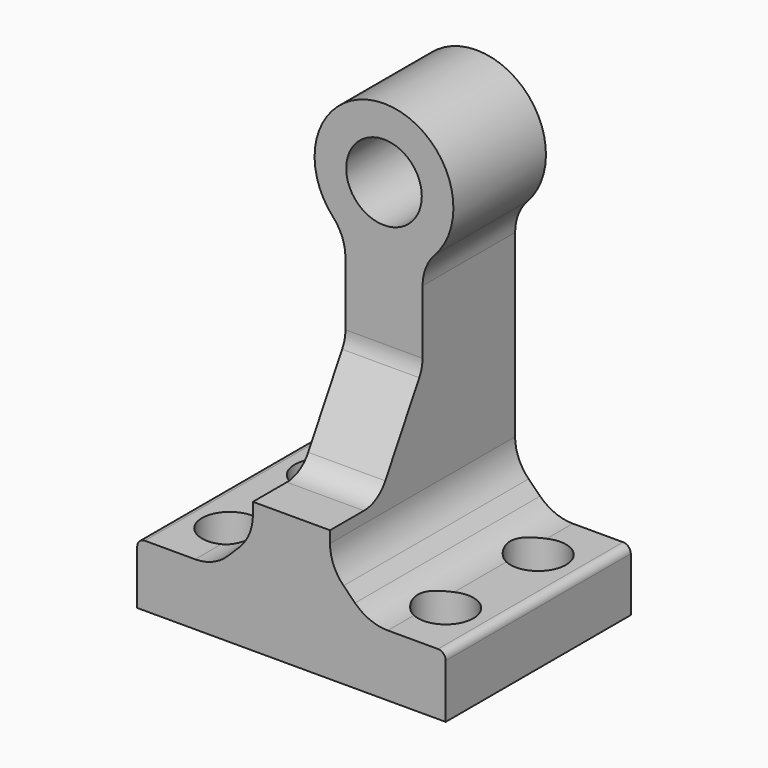
from build123d import *

# Parameters (mm, degrees)
F0_R          = 6.223
F1_DEPTH      = 19.05
F2_SIZE       = 6.35
F4_R          = 7.62
F3_R          = 2.413
F5_DEPTH      = 73.661
F6_R          = 4.572
F7_DEPTH      = 6.35
F7_DEPTH_BACK = 63.501
F8_R          = 1.27
F10_DEPTH     = 25.4
F11_R         = 5.08


# Not quite as in the source:
# - a pattern or mirror of a feature is missing from the dataset's text; its kind, count and spacing are read off the source's solid


with BuildPart() as f1:
    # F0 (on Front) → F1 (new body, symmetric)
    with BuildSketch(Plane.XZ):
        with BuildLine():
            Line((-25.4, 10.16), (-25.4, 0))
            Line((-25.4, 0), (25.4, 0))
            Line((25.4, 0), (25.4, 10.16))
            Line((25.4, 10.16), (6.35, 10.16))
            Line((6.35, 10.16), (6.35, 52.7261902376))
            ThreePointArc((6.35, 52.7261902376), (0, 73.66), (-6.35, 52.7261902376))
            Line((-6.35, 52.7261902376), (-6.35, 10.16))
            Line((-6.35, 10.16), (-25.4, 10.16))
        make_face()
        with Locations((0, 62.23)):
            Circle(F0_R, mode=Mode.SUBTRACT)
    extrude(amount=F1_DEPTH, both=True)

    # F2
    f2_edges = [f1.edges().sort_by_distance(p)[0] for p in [
        (-6.35, 0, 10.16),
        (6.35, 0, 10.16),
    ]]
    chamfer(f2_edges, length=F2_SIZE)

    # F4
    f4_edges = [f1.edges().sort_by_distance(p)[0] for p in [
        (-6.35, 0, 52.72619),
        (-6.35, 0, 16.51),
        (-12.7, 0, 10.16),
        (12.7, 0, 10.16),
        (6.35, 0, 16.51),
        (6.35, 0, 52.72619),
    ]]
    fillet(f4_edges, radius=F4_R)

    # F3 (on face) → F5 (cut, through all)
    with BuildSketch(Plane(origin=(0, 0, 0), x_dir=(1, 0, 0), z_dir=(0, 0, -1))):
        with Locations((-17.78, 9.525)):
            Circle(F3_R)
        with Locations((-17.78, -9.525)):
            Circle(F3_R)
    f5 = extrude(amount=-F5_DEPTH, mode=Mode.SUBTRACT)

    # F5_copies: F5 across plane
    add(f5.mirror(Plane(origin=(0, 0, 0), x_dir=(0, 0, 1), z_dir=(1, 0, 0))), mode=Mode.SUBTRACT)

    # F6 (on face) → F7 (cut, two sides)
    with BuildSketch(Plane.XY.offset(10.16)) as f7_sk:
        with Locations((-17.78, 9.525)):
            Circle(F6_R)
        with Locations((-17.78, -9.525)):
            Circle(F6_R)
    f7 = extrude(amount=-F7_DEPTH, mode=Mode.SUBTRACT) + extrude(f7_sk.sketch, amount=F7_DEPTH_BACK, mode=Mode.SUBTRACT)

    # F7_copies: F7 across plane
    add(f7.mirror(Plane(origin=(2e-06, 0, 0), x_dir=(0, 0, 1), z_dir=(1, 0, 0))), mode=Mode.SUBTRACT)

    # F8
    f8_edges = [f1.edges().sort_by_distance(p)[0] for p in [
        (-25.4, 0, 10.16),
        (25.4, 0, 10.16),
    ]]
    fillet(f8_edges, radius=F8_R)

    # F9 (on Right) → F10 (cut, symmetric)
    with BuildSketch(Plane.YZ):
        Polygon((0, 37.4132022262), (0, 76.8906995654), (-23.6530974507, 76.8906995654), (-23.6530974507, 21.59), (-9.1355300647, 21.59), align=None)
    extrude(amount=F10_DEPTH, both=True, mode=Mode.SUBTRACT)

    # F11
    f11_edges = [f1.edges().sort_by_distance(p)[0] for p in [
        (0, 0, 37.413202),
        (0, -9.13553, 21.59),
    ]]
    fillet(f11_edges, radius=F11_R)


solid = f1.part
